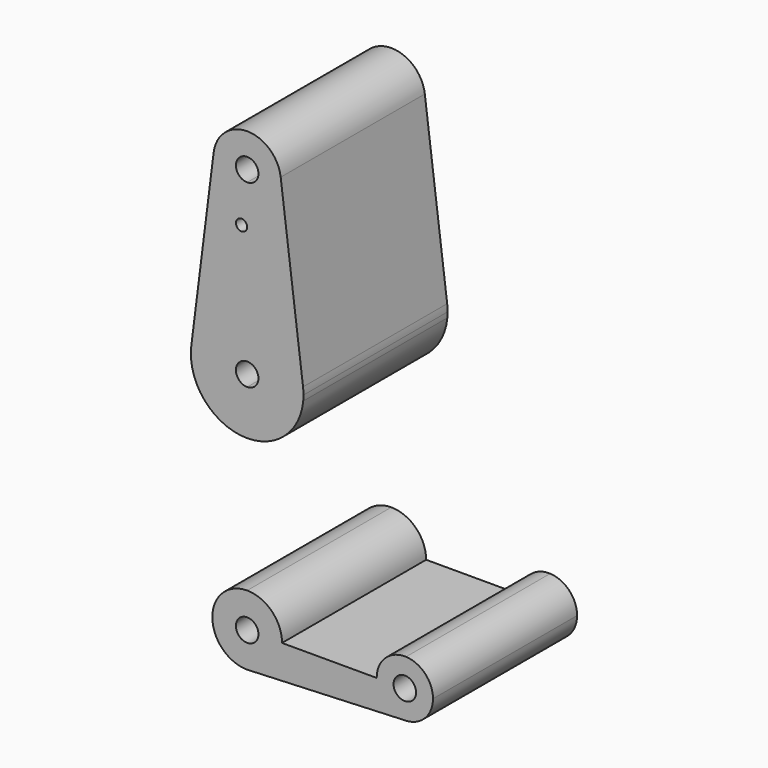
from build123d import *

# Parameters (mm, degrees)
F1_DEPTH = 50.8
F0_R     = 1.5875


with BuildPart() as f1:
    # F0 (on Front) → F1 (new body)
    with BuildSketch(Plane.XZ):
        with BuildLine():
            Line((3.175, 0), (9.8263469772, 0))
            ThreePointArc((9.8263469772, 0), (6.9482765818, 6.9482765818), (0, 9.8263469772))
            Line((0, 9.8263469772), (0, 3.175))
            ThreePointArc((0, 3.175), (2.2450640303, 2.2450640303), (3.175, 0))
        make_face()
        with BuildLine():
            Line((36.5125, 0), (9.8263469772, 0))
            ThreePointArc((9.8263469772, 0), (7.2359425088, -6.6481750072), (0.8304849282, -9.7911893915))
            Line((0.8304849282, -9.7911893915), (44.7857238654, -7.930396947))
            ThreePointArc((44.7857238654, -7.930396947), (38.9573185934, -5.7301271553), (36.5125, 0))
        make_face()
        with BuildLine():
            ThreePointArc((0.8304849282, -9.7911893915), (7.2359425088, -6.6481750072), (9.8263469772, 0))
            Line((9.8263469772, 0), (3.175, 0))
            ThreePointArc((3.175, 0), (-2.2450640303, -2.2450640303), (0, 3.175))
            Line((0, 3.175), (0, 9.8263469772))
            ThreePointArc((0, 9.8263469772), (-9.8263469772, 0), (0, -9.8263469772))
            Line((0, -9.8263469772), (0.8304849282, -9.7911893915))
        make_face()
        with BuildLine():
            ThreePointArc((0, -9.8263469772), (0.4156143861, -9.8175536463), (0.8304849282, -9.7911893915))
            Line((0.8304849282, -9.7911893915), (0, -9.8263469772))
        make_face()
        with BuildLine():
            ThreePointArc((44.7857238654, 7.930396947), (38.9573185934, 5.7301271553), (36.5125, 0))
            ThreePointArc((36.5125, 0), (38.9573185934, -5.7301271553), (44.7857238654, -7.930396947))
            ThreePointArc((44.7857238654, -7.930396947), (50.1801271553, -5.4926814066), (52.3875, 0))
            ThreePointArc((52.3875, 0), (50.1801271553, 5.4926814066), (44.7857238654, 7.930396947))
        make_face()
        with BuildLine():
            ThreePointArc((47.625, 0), (44.45, -3.175), (41.275, 0))
            ThreePointArc((41.275, 0), (44.45, 3.175), (47.625, 0))
        make_face(mode=Mode.SUBTRACT)
    extrude(amount=F1_DEPTH)


with BuildPart() as f1b:
    # F0 (on Front) → F1, piece 2 (new body)
    with BuildSketch(Plane.XZ):
        with BuildLine():
            ThreePointArc((-15.8028158025, 61.9878367443), (-10.677313176, 51.7522083632), (0, 47.625))
            Line((0, 47.625), (0, 60.325))
            ThreePointArc((0, 60.325), (-3.175, 63.5), (0, 66.675))
            Line((0, 66.675), (0, 79.375))
            ThreePointArc((0, 79.375), (-10.5003255158, 75.40625), (-15.7504882737, 65.484375))
            ThreePointArc((-15.7504882737, 65.484375), (-15.8732225611, 63.7375511007), (-15.8028158025, 61.9878367443))
        make_face()
        with BuildLine():
            Line((0, 60.325), (0, 47.625))
            ThreePointArc((0, 47.625), (10.677313176, 51.7522083632), (15.8028158025, 61.9878367443))
            ThreePointArc((15.8028158025, 61.9878367443), (15.8569436819, 62.7430574212), (15.875, 63.5))
            ThreePointArc((15.875, 63.5), (15.8438414904, 64.4941387366), (15.7504882737, 65.484375))
            ThreePointArc((15.7504882737, 65.484375), (10.5003255158, 75.40625), (0, 79.375))
            Line((0, 79.375), (0, 66.675))
            ThreePointArc((0, 66.675), (2.2450640303, 65.7450640303), (3.175, 63.5))
            ThreePointArc((3.175, 63.5), (2.2450640303, 61.2549359697), (0, 60.325))
        make_face()
        with BuildLine():
            Line((-9.4502929642, 115.490625), (-15.7504882737, 65.484375))
            ThreePointArc((-15.7504882737, 65.484375), (-10.5003255158, 75.40625), (0, 79.375))
            Line((0, 79.375), (0, 100.0252))
            Line((0, 100.0252), (0, 104.775))
            ThreePointArc((0, 104.775), (-7.14375, 107.9998046905), (-9.4502929642, 115.490625))
        make_face()
        with Locations((-1.5875, 100.0252)):
            Circle(F0_R, mode=Mode.SUBTRACT)
        with BuildLine():
            Line((0, 100.0252), (0, 79.375))
            ThreePointArc((0, 79.375), (10.5003255158, 75.40625), (15.7504882737, 65.484375))
            Line((15.7504882737, 65.484375), (9.4502929642, 115.490625))
            ThreePointArc((9.4502929642, 115.490625), (9.5063048942, 114.896483242), (9.525, 114.3))
            ThreePointArc((9.525, 114.3), (6.7351920908, 107.5648079092), (0, 104.775))
            Line((0, 104.775), (0, 100.0252))
        make_face()
        with BuildLine():
            ThreePointArc((9.4502929642, 115.490625), (0, 123.825), (-9.4502929642, 115.490625))
            ThreePointArc((-9.4502929642, 115.490625), (-7.14375, 107.9998046905), (0, 104.775))
            ThreePointArc((0, 104.775), (6.7351920908, 107.5648079092), (9.525, 114.3))
            ThreePointArc((9.525, 114.3), (9.5063048942, 114.896483242), (9.4502929642, 115.490625))
        make_face()
        with BuildLine():
            ThreePointArc((3.175, 114.3), (2.2450640303, 112.0549359697), (0, 111.125))
            ThreePointArc((0, 111.125), (-2.2450640303, 116.5450640303), (3.175, 114.3))
        make_face(mode=Mode.SUBTRACT)
    extrude(amount=F1_DEPTH)


solid = Compound([f1.part, f1b.part])
